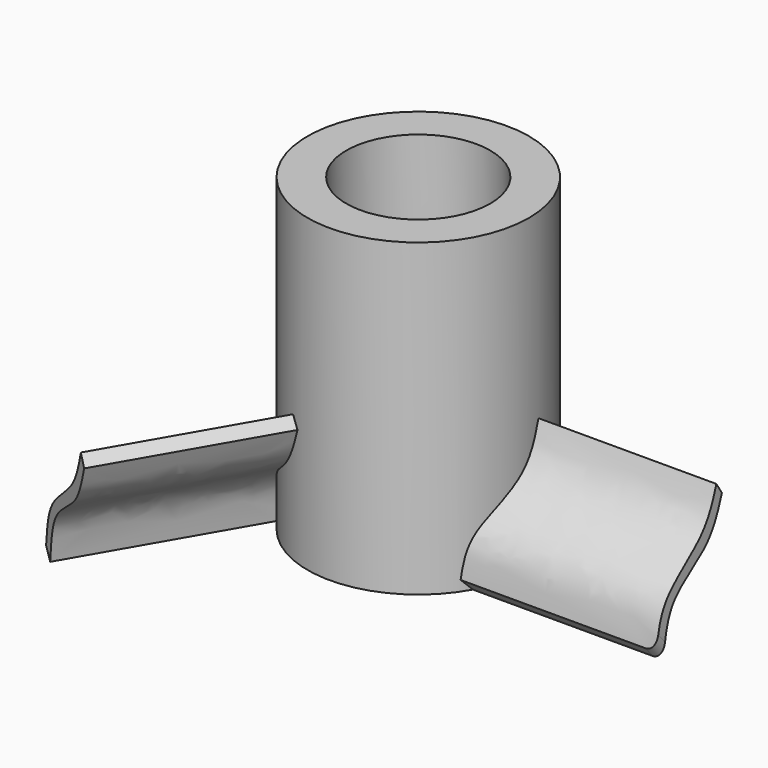
from build123d import *
from build123d import SkipClean  # not in build123d's __all__

# Parameters (mm, degrees)
F0_R            = 12.7
F1_DEPTH        = 35.56
F2_R            = 8.255
F3_DEPTH        = 9.525
F4_R            = 2.667
F5_DEPTH        = 254
F9_DEPTH        = 25.4
F9_COPIES_COUNT = 3
F10_R           = 1.27
F6_R            = 8.255
F6_R_2          = 2.667
F11_DEPTH       = 15.748


# Not quite as in the source:
# - a pattern or mirror of a feature is missing from the dataset's text; its kind, count and spacing are read off the source's solid
# - a feature names something its author has since deleted; it is built from what else it names


with BuildPart() as f1:
    # F0 (on Top) → F1 (new body)
    with BuildSketch(Plane.XY):
        Circle(F0_R)
    extrude(amount=F1_DEPTH)

    # F2 (on face) → F3 (cut)
    with BuildSketch(Plane.XY.offset(35.56)):
        Circle(F2_R)
    extrude(amount=-F3_DEPTH, mode=Mode.SUBTRACT)

    # F4 (on face) → F5 (cut)
    with BuildSketch(Plane.XY.offset(26.035)):
        Circle(F4_R)
    extrude(amount=-F5_DEPTH, mode=Mode.SUBTRACT)

    # F8 (on offset) → F9 (join)
    with BuildSketch(Plane.YZ.offset(7.62)):
        with BuildLine():
            Line((-7.096601933, 1.1829776548), (-6.096, 0))
            add(Edge.make_bspline(
                [(-6.096, 0), (-5.8943346547, 1.9452293607), (-5.4834307395, 5.9087381092), (0.5997187932, 8.6736721856), (1.7285446911, 11.9368345808), (2.2646340076, 13.4865390137)],
                knots=[0, 0, 0, 0, 0.3360272787, 0.6846735329, 1, 1, 1, 1], degree=3))
            Line((2.2646340076, 13.4865390137), (1.47131423, 14.712578617))
            add(Edge.make_bspline(
                [(-7.096601933, 1.1829776548), (-6.9020267489, 2.8395199903), (-6.4802421103, 6.4304409685), (-0.1009646663, 10.0195226908), (0.978146166, 13.2405336059), (1.47131423, 14.712578617)],
                knots=[0, 0, 0, 0, 0.3174047687, 0.6880448619, 1, 1, 1, 1], degree=3))
        make_face()
    with SkipClean():  # cleaning this boolean's faces spoils the solid; the shape is the same uncleaned
        f9 = extrude(amount=F9_DEPTH)

    # F9_copies: F9 ×3 about axis
    f9_copies_axis = Axis((0, 0, 0), (0, 0, 1))
    for i in range(1, F9_COPIES_COUNT):
        add(f9.rotate(f9_copies_axis, i * 360 / F9_COPIES_COUNT), clean=False)

    # F10
    f10_edges = [f1.edges().sort_by_distance(p)[0] for p in [
        (33.02, -6.596301, 0.591489),
    ]]
    fillet(f10_edges, radius=F10_R)

    # F6 (on face) → F11 (cut)
    with BuildSketch(Plane(origin=(0, 0, 0), x_dir=(1, 0, 0), z_dir=(0, 0, -1))):
        Circle(F6_R)
        Circle(F6_R_2, mode=Mode.SUBTRACT)
    extrude(amount=-F11_DEPTH, mode=Mode.SUBTRACT)


solid = f1.part
